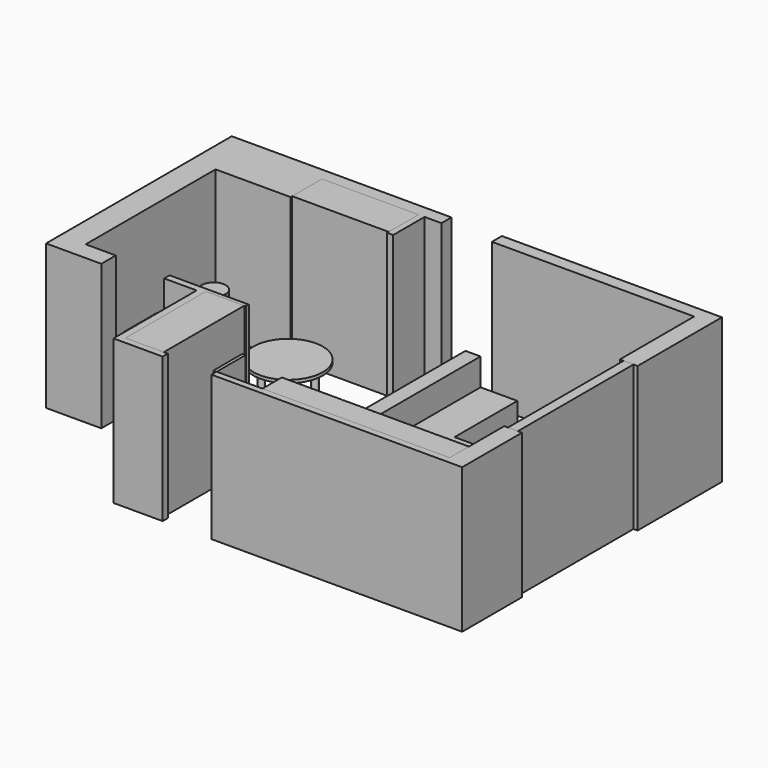
from build123d import *

# Parameters (mm, degrees)
F0_W      = 3351.6886112094
F0_H      = 207.362651825
F1_DEPTH  = 2400
F0_W_2    = 537.1888577938
F0_H_2    = 112.3662590981
F0_W_3    = 53.346157074
F0_H_3    = 600
F0_W_4    = 1250
F0_H_4    = 430
F0_W_5    = 550
F0_H_5    = 500
F2_DEPTH  = 900
F0_W_6    = 2000
F0_H_6    = 450
F0_R      = 50
F3_W      = 3100
F3_H      = 400
F4_DEPTH  = 800
F0_W_7    = 600
F0_H_7    = 650
F5_DEPTH  = 1900
F0_W_8    = 250
F0_H_8    = 2100
F6_DEPTH  = 900
F7_DEPTH  = 450
F0_W_9    = 350
F0_H_9    = 350
F8_DEPTH  = 910
F9_DEPTH  = 750
F10_DEPTH = 910
F11_W     = 450
F11_H     = 60
F12_DEPTH = 1000
F0_W_10   = 164.1221046448
F0_H_10   = 2394.7671353817
F13_DEPTH = 2400
F0_R_2    = 575
F14_DEPTH = 750
F15_DEPTH = 700
F17_DEPTH = 400
F0_R_3    = 150
F18_W     = 600
F18_H     = 600
F19_DEPTH = 25
F18_W_2   = 3100
F18_H_2   = 100
F20_DEPTH = 30
F21_W     = 10
F21_H     = 800
F22_DEPTH = 10
F23_W     = 700
F23_H     = 600
F24_DEPTH = 60
F0_W_11   = 1600
F0_H_11   = 616.584777832
F25_DEPTH = 2400
F0_R_4    = 200
F26_DEPTH = 1000
F0_W_12   = 450
F0_H_12   = 1400
F0_W_13   = 50
F0_H_13   = 1280
F27_DEPTH = 500
F28_DEPTH = 1300


# Not quite as in the source:
# - a feature names something its author has since deleted; it is built from what else it names


with BuildPart() as f1:
    # F0 (on Top) → F1 (new body)
    with BuildSketch(Plane.XY):
        Polygon((5332.8738090396, 2704.7533988953), (5394.4396972656, 2704.7533988953), (5558.5618019104, 2704.7533988953), (5626.5387535095, 2704.7533988953), (5626.5387535095, 4450.9944915771), (5332.8738090396, 4450.9944915771), (5332.8738090396, 4243.6318397522), align=None)
        with Locations((3657.0295034349, 4347.3131656647)):
            Rectangle(F0_W, F0_H)
    extrude(amount=F1_DEPTH)


with BuildPart() as f1b:
    # F0 (on Top) → F1, piece 2 (new body)
    with BuildSketch(Plane.XY):
        Polygon((5332.8738090396, -222.1663832664), (5332.8738090396, -822.1663832664), (2232.8738090396, -822.1663832664), (1474.7484922409, -822.1663832664), (1474.7484922409, -928.7706017494), (5626.5387535095, -928.7706017494), (5626.5387535095, 309.9862635136), (5558.5618019104, 309.9862635136), (5394.4396972656, 309.9862635136), (5332.8738090396, 309.9862635136), align=None)
    extrude(amount=F1_DEPTH)


with BuildPart() as f1c:
    # F0 (on Top) → F1, piece 3 (new body)
    with BuildSketch(Plane.XY):
        Polygon((597.9725122452, -822.1663832664), (-37.1261909604, -822.1663832664), (-37.1261909604, -26.347534731), (-37.1261909604, 845.5312275887), (-37.1261909604, 905.5312275887), (-150.5666673183, 905.5312275887), (-150.5666673183, 793.1649684906), (-150.5666673183, -928.7706017494), (664.8011207581, -928.7706017494), (664.8011207581, -822.1663832664), align=None)
        with Locations((-419.1610962152, 849.3480980396)):
            Rectangle(F0_W_2, F0_H_2)
        Polygon((-37.1261909604, 845.5312275887), (597.9725122452, 845.5312275887), (624.0934729576, 845.5312275887), (624.0934729576, 905.5312275887), (597.9725122452, 905.5312275887), (-37.1261909604, 905.5312275887), align=None)
    extrude(amount=F1_DEPTH)


with BuildPart() as f1d:
    # F0 (on Top) → F1, piece 4 (new body)
    with BuildSketch(Plane.XY):
        with Locations((1448.0754137039, -522.1663832664)):
            Rectangle(F0_W_3, F0_H_3)
    extrude(amount=F1_DEPTH)


with BuildPart() as f1e:
    # F0 (on Top) → F1, piece 5 (new body)
    with BuildSketch(Plane.XY):
        Polygon((865.7621264458, 4243.6318397522), (1145.4427242279, 4243.6318397522), (1145.4427242279, 4450.9944915771), (-2494.3199157715, 4450.9944915771), (-2494.3199157715, 605.3053736687), (-1579.2272090912, 605.3053736687), (-1579.2272090912, 905.5312275887), (-2078.3698558807, 905.5312275887), (-2078.3698558807, 3594.8448181152), (-834.2378735542, 3594.8448181152), (-834.2378735542, 3627.0470619202), (-834.2378735542, 4243.6318397522), (765.7621264458, 4243.6318397522), align=None)
        Polygon((865.7621264458, 3594.8448181152), (865.7621264458, 4243.6318397522), (765.7621264458, 4243.6318397522), (765.7621264458, 3627.0470619202), (765.7621264458, 3594.8448181152), align=None)
    extrude(amount=F1_DEPTH)


with BuildPart() as f2:
    # F0 (on Top) → F2 (new body)
    with BuildSketch(Plane.XY):
        Polygon((2232.8738090396, -822.1663832664), (5332.8738090396, -822.1663832664), (5332.8738090396, -222.1663832664), (4732.8738090396, -222.1663832664), (2232.8738090396, -222.1663832664), align=None)
        with Locations((2957.8738090396, -517.1663832664)):
            Rectangle(F0_W_4, F0_H_4, mode=Mode.SUBTRACT)
        with Locations((4757.8738090396, -522.1663832664)):
            Rectangle(F0_W_5, F0_H_5, mode=Mode.SUBTRACT)
    extrude(amount=F2_DEPTH)

    # F0 (on Top) → F8 (join)
    with BuildSketch(Plane.XY):
        with Locations((2957.8738090396, -517.1663832664)):
            Rectangle(F0_W_4, F0_H_4)
        with Locations((2957.8738090396, -507.1663832664)):
            Rectangle(F0_W_9, F0_H_9, mode=Mode.SUBTRACT)
        with Locations((3357.8738090396, -507.1663832664)):
            Rectangle(F0_W_9, F0_H_9, mode=Mode.SUBTRACT)
    extrude(amount=F8_DEPTH)

    # F0 (on Top) → F9 (join)
    with BuildSketch(Plane.XY):
        with Locations((3357.8738090396, -507.1663832664)):
            Rectangle(F0_W_9, F0_H_9)
        with Locations((2957.8738090396, -507.1663832664)):
            Rectangle(F0_W_9, F0_H_9)
    extrude(amount=F9_DEPTH)

    # F0 (on Top) → F10 (join)
    with BuildSketch(Plane.XY):
        with Locations((4757.8738090396, -522.1663832664)):
            Rectangle(F0_W_5, F0_H_5)
    extrude(amount=F10_DEPTH)

    # F18 (on face) → F19 (join)
    with BuildSketch(Plane(origin=(0, -222.1663832664, 0), x_dir=(-1, 0, 0), z_dir=(0, 1, 0))):
        with Locations((-4832.8738090396, 500)):
            Rectangle(F18_W, F18_H)
        with Locations((-4032.8738090396, 500)):
            Rectangle(F18_W, F18_H)
    extrude(amount=F19_DEPTH)

    # F18 (on face) → F20 (cut)
    with BuildSketch(Plane(origin=(0, -222.1663832664, 0), x_dir=(-1, 0, 0), z_dir=(0, 1, 0))):
        with Locations((-3782.8738090396, 50)):
            Rectangle(F18_W_2, F18_H_2)
    extrude(amount=-F20_DEPTH, mode=Mode.SUBTRACT)


with BuildPart() as f2b:
    # F0 (on Top) → F2, piece 2 (new body)
    with BuildSketch(Plane.XY):
        with Locations((3647.4789381027, 902.8336167336)):
            Rectangle(F0_W_6, F0_H_6)
    extrude(amount=F2_DEPTH)


with BuildPart() as f2c:
    # F0 (on Top) → F2, piece 3 (new body)
    with BuildSketch(Plane.XY):
        with Locations((1847.4789381027, 902.8336167336)):
            Circle(F0_R)
    extrude(amount=F2_DEPTH)


with BuildPart() as f4:
    # F3 (on face) → F4 (new body)
    with BuildSketch(Plane.XY.offset(2400)):
        with Locations((3782.8738090396, -622.1663832664)):
            Rectangle(F3_W, F3_H)
    extrude(amount=-F4_DEPTH)

    # F21 (on face) → F22 (cut)
    with BuildSketch(Plane(origin=(0, -422.1663832664, 0), x_dir=(-1, 0, 0), z_dir=(0, 1, 0))):
        with Locations((-2737.8738090396, 2000)):
            Rectangle(F21_W, F21_H)
        with Locations((-3247.8738090396, 2000)):
            Rectangle(F21_W, F21_H)
        with Locations((-3757.8738090396, 2000)):
            Rectangle(F21_W, F21_H)
        with Locations((-4267.8738090396, 2000)):
            Rectangle(F21_W, F21_H)
        with Locations((-4777.8738090396, 2000)):
            Rectangle(F21_W, F21_H)
    extrude(amount=-F22_DEPTH, mode=Mode.SUBTRACT)


with BuildPart() as f5:
    # F0 (on Top) → F5 (new body)
    with BuildSketch(Plane.XY):
        with Locations((1811.9415521622, -467.1663832664)):
            Rectangle(F0_W_7, F0_H_7)
    extrude(amount=F5_DEPTH)


with BuildPart() as f6:
    # F0 (on Top) → F6 (new body)
    with BuildSketch(Plane.XY):
        with Locations((1947.8738090396, 2843.6318397522)):
            Rectangle(F0_W_8, F0_H_8)
    extrude(amount=F6_DEPTH)

    # F0 (on Top) → F7 (join)
    with BuildSketch(Plane.XY):
        Polygon((2072.8738090396, 3893.6318397522), (2072.8738090396, 1793.6318397522), (3322.8738090396, 1793.6318397522), (3322.8738090396, 2593.6318397522), (2682.8738090396, 2593.6318397522), (2682.8738090396, 3893.6318397522), align=None)
    extrude(amount=F7_DEPTH)


with BuildPart() as f12:
    # F11 (on face) → F12 (new body)
    with BuildSketch(Plane(origin=(2647.4789381027, 0, 0), x_dir=(0, -1, 0), z_dir=(-1, 0, 0))):
        with Locations((-902.8336167336, 870)):
            Rectangle(F11_W, F11_H)
    extrude(amount=F12_DEPTH)


with BuildPart() as f13:
    # F0 (on Top) → F13 (new body)
    with BuildSketch(Plane.XY):
        with Locations((5476.500749588, 1507.3698312044)):
            Rectangle(F0_W_10, F0_H_10)
    extrude(amount=F13_DEPTH)


with BuildPart() as f14:
    # F0 (on Top) → F14 (new body)
    with BuildSketch(Plane.XY):
        with Locations((0, 2500.5469322205)):
            Circle(F0_R_2)
        with Locations((-247.4873734153, 2253.0595588052)):
            Circle(F0_R, mode=Mode.SUBTRACT)
        with Locations((247.4873734153, 2253.0595588052)):
            Circle(F0_R, mode=Mode.SUBTRACT)
        with Locations((-247.4873734153, 2748.0343056358)):
            Circle(F0_R, mode=Mode.SUBTRACT)
        with Locations((247.4873734153, 2748.0343056358)):
            Circle(F0_R, mode=Mode.SUBTRACT)
        with Locations((247.4873734153, 2748.0343056358)):
            Circle(F0_R)
        with Locations((247.4873734153, 2253.0595588052)):
            Circle(F0_R)
        with Locations((-247.4873734153, 2748.0343056358)):
            Circle(F0_R)
        with Locations((-247.4873734153, 2253.0595588052)):
            Circle(F0_R)
    extrude(amount=F14_DEPTH)


with BuildPart() as f15:
    # F0 (on Top) → F15 (new body)
    with BuildSketch(Plane.XY):
        with Locations((0, 2500.5469322205)):
            Circle(F0_R_2)
        with Locations((-247.4873734153, 2253.0595588052)):
            Circle(F0_R, mode=Mode.SUBTRACT)
        with Locations((247.4873734153, 2253.0595588052)):
            Circle(F0_R, mode=Mode.SUBTRACT)
        with Locations((-247.4873734153, 2748.0343056358)):
            Circle(F0_R, mode=Mode.SUBTRACT)
        with Locations((247.4873734153, 2748.0343056358)):
            Circle(F0_R, mode=Mode.SUBTRACT)
    extrude(amount=F15_DEPTH)


with BuildPart() as f14_1:
    add(f14.part)

    # F16: cut F15
    add(f15.part, mode=Mode.SUBTRACT)


with BuildPart() as f17:
    # F0 (on Top) → F17 (new body)
    with BuildSketch(Plane.XY):
        with BuildLine():
            ThreePointArc((3356.5598369582, 3718.6318397522), (3490.1661397403, 3245.7694746289), (3832.8738090396, 2893.6318397522))
            ThreePointArc((3832.8738090396, 2893.6318397522), (4175.5814783389, 3245.7694746289), (4309.187781121, 3718.6318397522))
            ThreePointArc((4309.187781121, 3718.6318397522), (3832.8738090396, 3839.3565699987), (3356.5598369582, 3718.6318397522))
        make_face()
    extrude(amount=F17_DEPTH)


with BuildPart() as f17b:
    # F0 (on Top) → F17, piece 2 (new body)
    with BuildSketch(Plane.XY):
        with Locations((4373.0506326787, 2080.4357423588)):
            Circle(F0_R_3)
    extrude(amount=F17_DEPTH)


with BuildPart() as f24:
    # F23 (on face) → F24 (new body)
    with BuildSketch(Plane.YZ.offset(-2078.3698558807)):
        with Locations((2026.7077445984, 500)):
            Rectangle(F23_W, F23_H)
    extrude(amount=F24_DEPTH)


with BuildPart() as f25:
    # F0 (on Top) → F25 (new body)
    with BuildSketch(Plane.XY):
        with Locations((-34.2378735542, 3935.3394508362)):
            Rectangle(F0_W_11, F0_H_11)
    extrude(amount=F25_DEPTH)


with BuildPart() as f25b:
    # F0 (on Top) → F25, piece 2 (new body)
    with BuildSketch(Plane.XY):
        Polygon((-37.1261909604, -26.347534731), (-37.1261909604, -822.1663832664), (597.9725122452, -822.1663832664), (597.9725122452, 845.5312275887), (-37.1261909604, 845.5312275887), align=None)
    extrude(amount=F25_DEPTH)


with BuildPart() as f26:
    # F0 (on Top) → F26 (new body)
    with BuildSketch(Plane.XY):
        with Locations((-1673.9757061005, 3049.9031543732)):
            Circle(F0_R_4)
    extrude(amount=F26_DEPTH)


with BuildPart() as f27:
    # F0 (on Top) → F27 (new body)
    with BuildSketch(Plane.XY):
        with Locations((5032.7116012573, 3143.6318397522)):
            Rectangle(F0_W_12, F0_H_12)
        with Locations((5031.8699836731, 3149.9679946899)):
            Rectangle(F0_W_13, F0_H_13, mode=Mode.SUBTRACT)
    extrude(amount=F27_DEPTH)


with BuildPart() as f28:
    # F0 (on Top) → F28 (new body)
    with BuildSketch(Plane.XY):
        with Locations((5031.8699836731, 3149.9679946899)):
            Rectangle(F0_W_13, F0_H_13)
    extrude(amount=F28_DEPTH)


solid = Compound([f1.part, f1b.part, f1c.part, f1d.part, f1e.part, f2.part, f2b.part, f2c.part, f4.part, f5.part, f6.part, f12.part, f13.part, f14_1.part, f17.part, f17b.part, f24.part, f25.part, f25b.part, f26.part, f27.part, f28.part])
